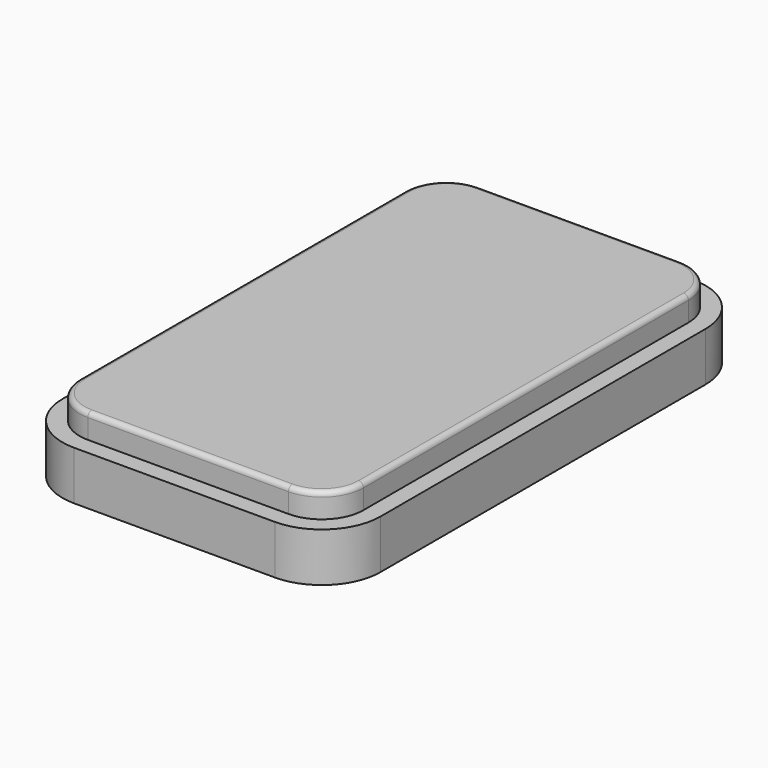
from build123d import *

# Parameters (mm, degrees)
F1_DEPTH = 5
F3_DEPTH = 10
F4_R     = 1


# Not quite as in the source:
# - a feature names something its author has since deleted; it is built from what else it names


with BuildPart() as f1:
    # F0 (on Top) → F1 (new body)
    with BuildSketch(Plane.XY):
        with BuildLine():
            Line((29, -41.5), (29, 41.5))
            ThreePointArc((29, 41.5), (26.5104076401, 47.5104076401), (20.5, 50))
            Line((20.5, 50), (-20.5, 50))
            ThreePointArc((-20.5, 50), (-26.5104076401, 47.5104076401), (-29, 41.5))
            Line((-29, 41.5), (-29, -41.5))
            ThreePointArc((-29, -41.5), (-26.5104076401, -47.5104076401), (-20.5, -50))
            Line((-20.5, -50), (20.5, -50))
            ThreePointArc((20.5, -50), (26.5104076401, -47.5104076401), (29, -41.5))
        make_face()
    extrude(amount=F1_DEPTH)

    # F2 (on Top) → F3 (join)
    with BuildSketch(Plane.XY):
        with BuildLine():
            ThreePointArc((32.5, 41.5), (28.9852813742, 49.9852813742), (20.5, 53.5))
            Line((20.5, 53.5), (-20.5, 53.5))
            ThreePointArc((-20.5, 53.5), (-28.9852813742, 49.9852813742), (-32.5, 41.5))
            Line((-32.5, 41.5), (-32.5, -41.5))
            ThreePointArc((-32.5, -41.5), (-28.9852813742, -49.9852813742), (-20.5, -53.5))
            Line((-20.5, -53.5), (20.5, -53.5))
            ThreePointArc((20.5, -53.5), (28.9852813742, -49.9852813742), (32.5, -41.5))
            Line((32.5, -41.5), (32.5, 41.5))
        make_face()
    extrude(amount=-F3_DEPTH)

    # F4
    f4_edges = [f1.edges().sort_by_distance(p)[0] for p in [
        (0, 50, 5),
        (-26.510408, 47.510408, 5),
        (-29, 0, 5),
        (-26.510408, -47.510408, 5),
        (0, -50, 5),
        (26.510408, -47.510408, 5),
        (29, 0, 5),
        (26.510408, 47.510408, 5),
    ]]
    fillet(f4_edges, radius=F4_R)


solid = f1.part
